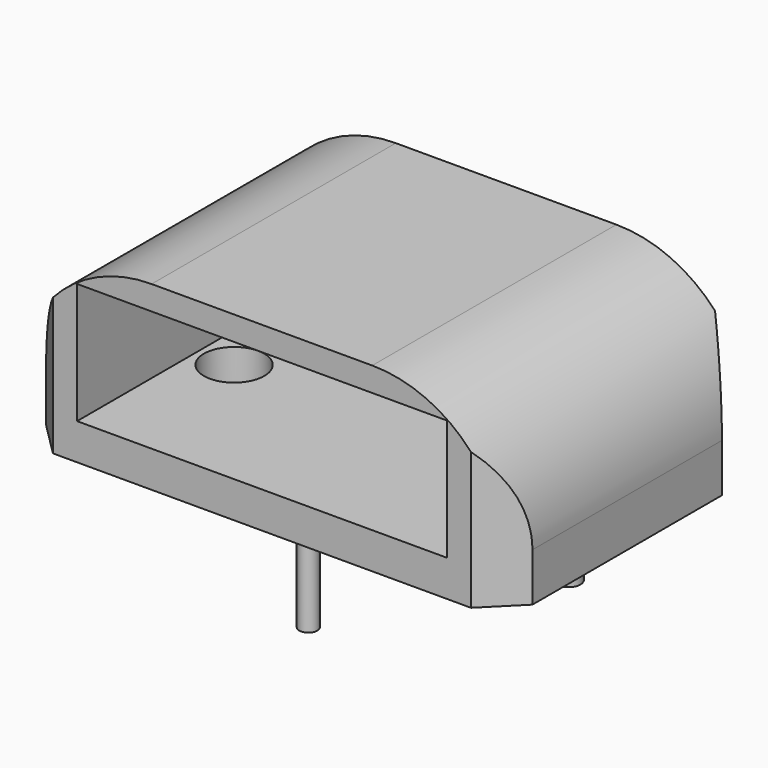
from build123d import *

# Parameters (mm, degrees)
F1_DEPTH  = 15
F2_W      = 30.607
F2_H      = 10
F3_DEPTH  = 25
F4_DEPTH  = 20
F6_DEPTH  = 9
F7_DEPTH  = 9
F8_R      = 11
F9_R      = 2.5
F10_DEPTH = 25


# Not quite as in the source:
# - a feature names something its author has since deleted; it is built from what else it names


with BuildPart() as f1:
    # F0 (on Top) → F1 (new body)
    with BuildSketch(Plane.XY):
        Polygon((37.435, 25.263), (2.828, 25.263), (0, 22.435), (0, 2.828), (2.828, 0), (37.435, 0), (40.263, 2.828), (40.263, 22.435), align=None)
    extrude(amount=F1_DEPTH)

    # F2 (on face) → F3 (cut)
    with BuildSketch(Plane.XZ):
        with Locations((20.1315, 8)):
            Rectangle(F2_W, F2_H)
    extrude(amount=-F3_DEPTH, mode=Mode.SUBTRACT)

    # F2 (on face) → F4 (cut)
    with BuildSketch(Plane.XZ):
        with Locations((20.1315, 8)):
            Rectangle(F2_W, F2_H)
    extrude(amount=-F4_DEPTH, mode=Mode.SUBTRACT)

    # F5 (on face) → F6 (join)
    with BuildSketch(Plane(origin=(0, 0, 0), x_dir=(1, 0, 0), z_dir=(0, 0, -1))):
        with BuildLine():
            ThreePointArc((12.1315, -20.463), (11.1315, -19.463), (10.1315, -20.463))
            Line((10.1315, -20.463), (12.1315, -20.463))
        make_face()
        with BuildLine():
            Line((12.1315, -20.463), (10.1315, -20.463))
            ThreePointArc((10.1315, -20.463), (11.1315, -21.463), (12.1315, -20.463))
        make_face()
        with BuildLine():
            Line((18.6315, -20.463), (21.6315, -20.463))
            ThreePointArc((21.6315, -20.463), (20.1315, -18.963), (18.6315, -20.463))
        make_face()
        with BuildLine():
            ThreePointArc((18.6315, -20.463), (20.1315, -21.963), (21.6315, -20.463))
            Line((21.6315, -20.463), (18.6315, -20.463))
        make_face()
        with BuildLine():
            ThreePointArc((28.1315, -20.463), (29.1315, -21.463), (30.1315, -20.463))
            Line((30.1315, -20.463), (28.1315, -20.463))
        make_face()
        with BuildLine():
            Line((28.1315, -20.463), (30.1315, -20.463))
            ThreePointArc((30.1315, -20.463), (29.1315, -19.463), (28.1315, -20.463))
        make_face()
    extrude(amount=F6_DEPTH)

    # F5 (on face) → F7 (join)
    with BuildSketch(Plane(origin=(0, 0, 0), x_dir=(1, 0, 0), z_dir=(0, 0, -1))):
        with BuildLine():
            Line((19.3815, -4.8), (20.8815, -4.8))
            ThreePointArc((20.8815, -4.8), (20.1315, -4.05), (19.3815, -4.8))
        make_face()
        with BuildLine():
            ThreePointArc((19.3815, -4.8), (20.1315, -5.55), (20.8815, -4.8))
            Line((20.8815, -4.8), (19.3815, -4.8))
        make_face()
    extrude(amount=F7_DEPTH)

    # F8
    f8_edges = [f1.edges().sort_by_distance(p)[0] for p in [
        (40.263, 12.6315, 15),
        (0, 12.6315, 15),
    ]]
    fillet(f8_edges, radius=F8_R)

    # F9 (on face) → F10 (cut)
    with BuildSketch(Plane.XY.offset(3)):
        with Locations((7.828, 12.5)):
            Circle(F9_R)
    extrude(amount=-F10_DEPTH, mode=Mode.SUBTRACT)


solid = f1.part
